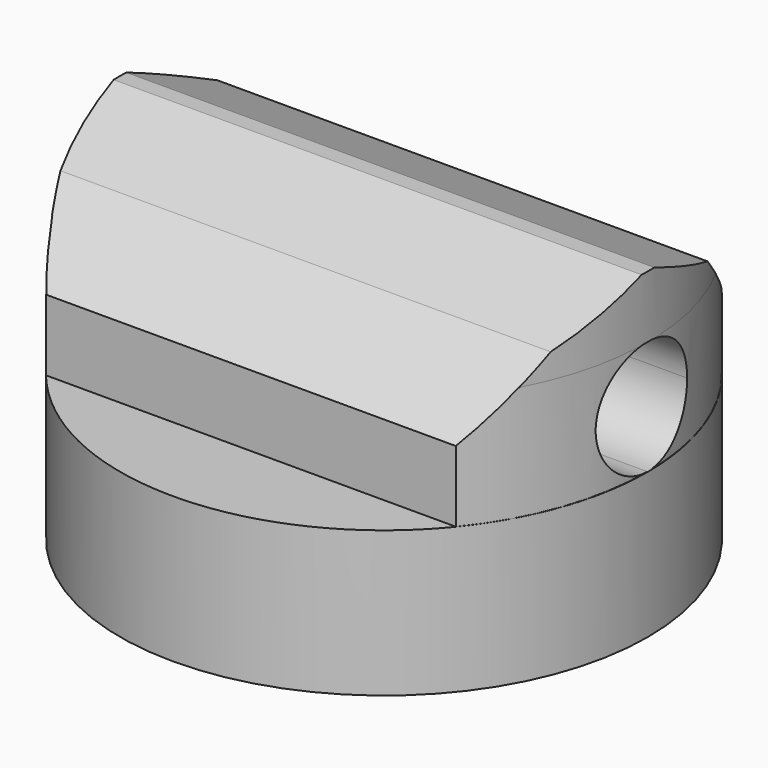
from build123d import *

# Parameters (mm, degrees)
F0_R         = 12.7
F0_R_2       = 6.25
F1_DEPTH     = 4
F3_R         = 12.7
F4_DEPTH     = 3
F7_DEPTH     = 5.5
F10_DEPTH    = 3
F11_R        = 2.74999
F12_T1_DEPTH = 45.8363262896
F13_SIZE     = 2.54


# Not quite as in the source:
# - a fillet or chamfer that OpenCascade refuses, or shapes differently, is made with other operations: its cross-section is extruded or revolved along the edge and cut away or added
# - a fillet or chamfer is up to 0.001 mm smaller than in the source, because OpenCascade refuses the exact size


with BuildPart() as f1:
    # F0 (on Top) → F1 (new body)
    with BuildSketch(Plane.XY):
        Circle(F0_R)
        Circle(F0_R_2, mode=Mode.SUBTRACT)
    extrude(amount=F1_DEPTH)

    # F3 (on offset) → F4 (join)
    with BuildSketch(Plane.XY.offset(4)):
        Circle(F3_R)
    extrude(amount=F4_DEPTH)

    # F6 (on offset) → F7 (join)
    with BuildSketch(Plane.XY.offset(7)):
        with BuildLine():
            Line((3.67872e-05, 2.75), (12.3864002526, 2.75))
            ThreePointArc((12.3864002526, 2.75), (11.4283726358, 5.5236330803), (9.8540587351, 8))
            Line((9.8540587351, 8), (-9.8539683968, 8))
            ThreePointArc((-9.8539683968, 8), (-11.4266416959, 5.5228386705), (-12.3863266781, 2.75))
            Line((-12.3863266781, 2.75), (-4.0361126885, 2.75))
            Line((-4.0361126885, 2.75), (3.67872e-05, 2.75))
        make_face()
        with BuildLine():
            Line((12.3864002526, -2.75), (3.67872e-05, -2.75))
            Line((3.67872e-05, -2.75), (-4.0361126885, -2.75))
            Line((-4.0361126885, -2.75), (-12.3863266781, -2.75))
            ThreePointArc((-12.3863266781, -2.75), (-11.4266416959, -5.5228386705), (-9.8539683968, -8))
            Line((-9.8539683968, -8), (9.8540587351, -8))
            ThreePointArc((9.8540587351, -8), (11.4283726358, -5.5236330803), (12.3864002526, -2.75))
        make_face()
    extrude(amount=F7_DEPTH)

    # F9 (on offset) → F10 (join)
    with BuildSketch(Plane.XY.offset(12.5)):
        with BuildLine():
            Line((-9.8539683968, -8), (9.8540587351, -8))
            ThreePointArc((9.8540587351, -8), (12.7066576307, 0), (9.8540587351, 8))
            Line((9.8540587351, 8), (-9.8539683968, 8))
            ThreePointArc((-9.8539683968, 8), (-12.7123228833, 0), (-9.8539683968, -8))
        make_face()
    extrude(amount=F10_DEPTH)

    # F11 (radius 2.75 in the source; OpenCascade refuses exactly that, so slightly less here)
    f11_edges = [f1.edges().sort_by_distance(p)[0] for p in [
        (3.7e-05, -2.75, 7),
        (3.7e-05, -2.75, 12.5),
        (3.7e-05, 2.75, 12.5),
        (3.7e-05, 2.75, 7),
    ]]
    fillet(f11_edges, radius=F11_R)

    # F12: chamfer of 5.08 on 2 edges, made by hand

    # F12_s2 → F12_t1 (cut)
    with BuildSketch(Plane.YZ.offset(-22.9181179756)):
        Polygon((8, 10.42), (2.92, 15.5), (8, 15.5), align=None)
        Polygon((-8, 10.42), (-2.92, 15.5), (-8, 15.5), align=None)
    extrude(amount=F12_T1_DEPTH, mode=Mode.SUBTRACT)

    # F13
    f13_edges = [f1.edges().sort_by_distance(p)[0] for p in [
        (-0.002558, 2.92, 15.5),
        (-0.002558, -2.92, 15.5),
    ]]
    chamfer(f13_edges, length=F13_SIZE)


solid = f1.part
